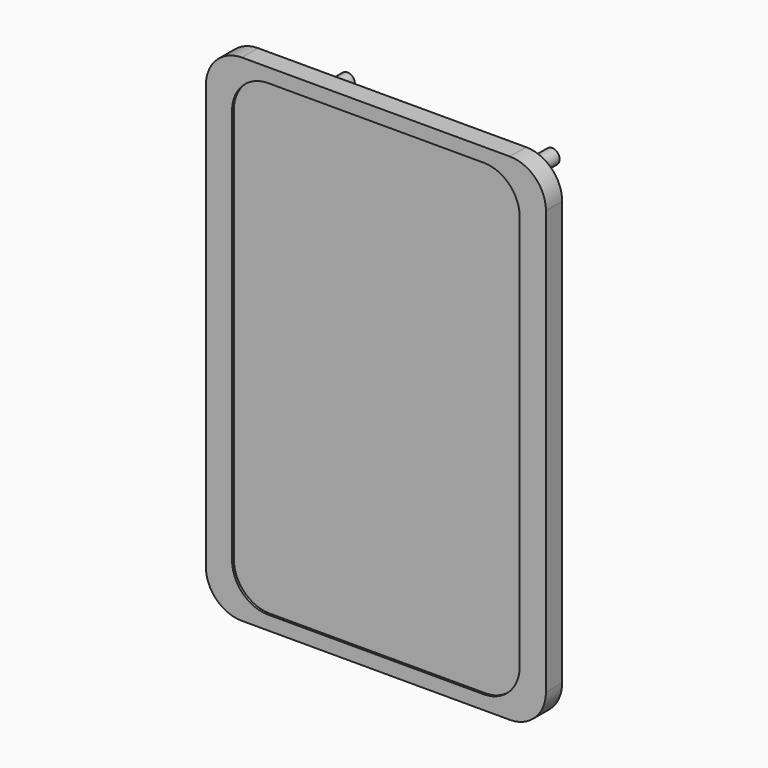
from build123d import *

# Parameters (mm, degrees)
F0_R     = 2.5
F0_W     = 0.95
F0_H     = 30
F0_R_2   = 1.2
F0_R_3   = 0.825
F1_DEPTH = 2
F2_DEPTH = 2
F3_DEPTH = 2.25
F4_DEPTH = 8
F5_DEPTH = 5.5
F6_DEPTH = 3.9


# Not quite as in the source:
# - a feature names something its author has since deleted; it is built from what else it names


with BuildPart() as f1:
    # F0 (on Front) → F1 (new body)
    with BuildSketch(Plane.XZ):
        with BuildLine():
            Line((0, 25), (0, -25))
            Line((0, -25), (11, -25))
            ThreePointArc((11, -25), (13.8284271247, -23.8284271247), (15, -21))
            Line((15, -21), (15, -15))
            Line((15, -15), (15, 15))
            Line((15, 15), (15, 21))
            ThreePointArc((15, 21), (13.8284271247, 23.8284271247), (11, 25))
            Line((11, 25), (0, 25))
        make_face()
        with Locations((11.35, -16.05)):
            Circle(F0_R, mode=Mode.SUBTRACT)
        with Locations((11.35, 22.2)):
            Circle(F0_R, mode=Mode.SUBTRACT)
        with BuildLine():
            Line((-11, -25), (0, -25))
            Line((0, -25), (0, 25))
            Line((0, 25), (-11, 25))
            ThreePointArc((-11, 25), (-13.8284271247, 23.8284271247), (-15, 21))
            Line((-15, 21), (-15, 15))
            Line((-15, 15), (-15, -15))
            Line((-15, -15), (-15, -21))
            ThreePointArc((-15, -21), (-13.8284271247, -23.8284271247), (-11, -25))
        make_face()
        with Locations((-11.35, -16.05)):
            Circle(F0_R, mode=Mode.SUBTRACT)
        with Locations((-11.35, 22.2)):
            Circle(F0_R, mode=Mode.SUBTRACT)
        with BuildLine():
            Line((0, -27.5), (0, -25.95))
            Line((0, -25.95), (-11.95, -25.95))
            ThreePointArc((-11.95, -25.95), (-14.7784271247, -24.7784271247), (-15.95, -21.95))
            Line((-15.95, -21.95), (-15.95, -15))
            Line((-15.95, -15), (-15.95, 15))
            Line((-15.95, 15), (-15.95, 21.95))
            ThreePointArc((-15.95, 21.95), (-14.7784271247, 24.7784271247), (-11.95, 25.95))
            Line((-11.95, 25.95), (0, 25.95))
            Line((0, 25.95), (0, 27.5))
            Line((0, 27.5), (-14.8588332385, 27.5))
            ThreePointArc((-14.8588332385, 27.5), (-17.6872603632, 26.3284271247), (-18.8588332385, 23.5))
            Line((-18.8588332385, 23.5), (-18.8588332385, -23.5))
            ThreePointArc((-18.8588332385, -23.5), (-17.6872603632, -26.3284271247), (-14.8588332385, -27.5))
            Line((-14.8588332385, -27.5), (0, -27.5))
        make_face()
        with BuildLine():
            ThreePointArc((15.95, -21.95), (14.7784271247, -24.7784271247), (11.95, -25.95))
            Line((11.95, -25.95), (0, -25.95))
            Line((0, -25.95), (0, -27.5))
            Line((0, -27.5), (14.8588332385, -27.5))
            ThreePointArc((14.8588332385, -27.5), (17.6872603632, -26.3284271247), (18.8588332385, -23.5))
            Line((18.8588332385, -23.5), (18.8588332385, 23.5))
            ThreePointArc((18.8588332385, 23.5), (17.6872603632, 26.3284271247), (14.8588332385, 27.5))
            Line((14.8588332385, 27.5), (0, 27.5))
            Line((0, 27.5), (0, 25.95))
            Line((0, 25.95), (11.95, 25.95))
            ThreePointArc((11.95, 25.95), (14.7784271247, 24.7784271247), (15.95, 21.95))
            Line((15.95, 21.95), (15.95, 15))
            Line((15.95, 15), (15.95, -15))
            Line((15.95, -15), (15.95, -21.95))
        make_face()
        with Locations((15.475, 0)):
            Rectangle(F0_W, F0_H)
        with Locations((-15.475, 0)):
            Rectangle(F0_W, F0_H)
        with BuildLine():
            Line((-11, 25), (0, 25))
            Line((0, 25), (0, 25.95))
            Line((0, 25.95), (-11.95, 25.95))
            ThreePointArc((-11.95, 25.95), (-14.7784271247, 24.7784271247), (-15.95, 21.95))
            Line((-15.95, 21.95), (-15.95, 15))
            Line((-15.95, 15), (-15, 15))
            Line((-15, 15), (-15, 21))
            ThreePointArc((-15, 21), (-13.8284271247, 23.8284271247), (-11, 25))
        make_face()
        with BuildLine():
            Line((0, 25.95), (0, 25))
            Line((0, 25), (11, 25))
            ThreePointArc((11, 25), (13.8284271247, 23.8284271247), (15, 21))
            Line((15, 21), (15, 15))
            Line((15, 15), (15.95, 15))
            Line((15.95, 15), (15.95, 21.95))
            ThreePointArc((15.95, 21.95), (14.7784271247, 24.7784271247), (11.95, 25.95))
            Line((11.95, 25.95), (0, 25.95))
        make_face()
        with BuildLine():
            Line((0, -25.95), (11.95, -25.95))
            ThreePointArc((11.95, -25.95), (14.7784271247, -24.7784271247), (15.95, -21.95))
            Line((15.95, -21.95), (15.95, -15))
            Line((15.95, -15), (15, -15))
            Line((15, -15), (15, -21))
            ThreePointArc((15, -21), (13.8284271247, -23.8284271247), (11, -25))
            Line((11, -25), (0, -25))
            Line((0, -25), (0, -25.95))
        make_face()
        with BuildLine():
            Line((-11.95, -25.95), (0, -25.95))
            Line((0, -25.95), (0, -25))
            Line((0, -25), (-11, -25))
            ThreePointArc((-11, -25), (-13.8284271247, -23.8284271247), (-15, -21))
            Line((-15, -21), (-15, -15))
            Line((-15, -15), (-15.95, -15))
            Line((-15.95, -15), (-15.95, -21.95))
            ThreePointArc((-15.95, -21.95), (-14.7784271247, -24.7784271247), (-11.95, -25.95))
        make_face()
        with Locations((11.35, -16.05)):
            Circle(F0_R)
        with Locations((11.35, -16.05)):
            Circle(F0_R_2, mode=Mode.SUBTRACT)
        with Locations((-11.35, -16.05)):
            Circle(F0_R)
        with Locations((-11.35, -16.05)):
            Circle(F0_R_2, mode=Mode.SUBTRACT)
        with Locations((11.35, 22.2)):
            Circle(F0_R)
        with Locations((11.35, 22.2)):
            Circle(F0_R_2, mode=Mode.SUBTRACT)
        with Locations((-11.35, 22.2)):
            Circle(F0_R)
        with Locations((-11.35, 22.2)):
            Circle(F0_R_2, mode=Mode.SUBTRACT)
        with Locations((-11.35, -16.05)):
            Circle(F0_R_2)
        with Locations((-11.35, -16.05)):
            Circle(F0_R_3, mode=Mode.SUBTRACT)
        with Locations((11.35, 22.2)):
            Circle(F0_R_2)
        with Locations((11.35, 22.2)):
            Circle(F0_R_3, mode=Mode.SUBTRACT)
        with Locations((-11.35, 22.2)):
            Circle(F0_R_2)
        with Locations((-11.35, 22.2)):
            Circle(F0_R_3, mode=Mode.SUBTRACT)
        with Locations((11.35, -16.05)):
            Circle(F0_R_2)
        with Locations((11.35, -16.05)):
            Circle(F0_R_3, mode=Mode.SUBTRACT)
        with Locations((-11.35, -16.05)):
            Circle(F0_R_3)
        with Locations((11.35, -16.05)):
            Circle(F0_R_3)
        with Locations((11.35, 22.2)):
            Circle(F0_R_3)
        with Locations((-11.35, 22.2)):
            Circle(F0_R_3)
    extrude(amount=F1_DEPTH)

    # F0 (on Front) → F2 (join)
    with BuildSketch(Plane.XZ):
        with BuildLine():
            Line((0, -25.95), (11.95, -25.95))
            ThreePointArc((11.95, -25.95), (14.7784271247, -24.7784271247), (15.95, -21.95))
            Line((15.95, -21.95), (15.95, -15))
            Line((15.95, -15), (15, -15))
            Line((15, -15), (15, -21))
            ThreePointArc((15, -21), (13.8284271247, -23.8284271247), (11, -25))
            Line((11, -25), (0, -25))
            Line((0, -25), (0, -25.95))
        make_face()
        with Locations((15.475, 0)):
            Rectangle(F0_W, F0_H)
        with BuildLine():
            Line((0, 25.95), (0, 25))
            Line((0, 25), (11, 25))
            ThreePointArc((11, 25), (13.8284271247, 23.8284271247), (15, 21))
            Line((15, 21), (15, 15))
            Line((15, 15), (15.95, 15))
            Line((15.95, 15), (15.95, 21.95))
            ThreePointArc((15.95, 21.95), (14.7784271247, 24.7784271247), (11.95, 25.95))
            Line((11.95, 25.95), (0, 25.95))
        make_face()
        with BuildLine():
            Line((-11.95, -25.95), (0, -25.95))
            Line((0, -25.95), (0, -25))
            Line((0, -25), (-11, -25))
            ThreePointArc((-11, -25), (-13.8284271247, -23.8284271247), (-15, -21))
            Line((-15, -21), (-15, -15))
            Line((-15, -15), (-15.95, -15))
            Line((-15.95, -15), (-15.95, -21.95))
            ThreePointArc((-15.95, -21.95), (-14.7784271247, -24.7784271247), (-11.95, -25.95))
        make_face()
        with Locations((-15.475, 0)):
            Rectangle(F0_W, F0_H)
        with BuildLine():
            Line((-11, 25), (0, 25))
            Line((0, 25), (0, 25.95))
            Line((0, 25.95), (-11.95, 25.95))
            ThreePointArc((-11.95, 25.95), (-14.7784271247, 24.7784271247), (-15.95, 21.95))
            Line((-15.95, 21.95), (-15.95, 15))
            Line((-15.95, 15), (-15, 15))
            Line((-15, 15), (-15, 21))
            ThreePointArc((-15, 21), (-13.8284271247, 23.8284271247), (-11, 25))
        make_face()
    extrude(amount=-F2_DEPTH)

    # F0 (on Front) → F3 (join)
    with BuildSketch(Plane.XZ):
        with BuildLine():
            ThreePointArc((15.95, -21.95), (14.7784271247, -24.7784271247), (11.95, -25.95))
            Line((11.95, -25.95), (0, -25.95))
            Line((0, -25.95), (0, -27.5))
            Line((0, -27.5), (14.8588332385, -27.5))
            ThreePointArc((14.8588332385, -27.5), (17.6872603632, -26.3284271247), (18.8588332385, -23.5))
            Line((18.8588332385, -23.5), (18.8588332385, 23.5))
            ThreePointArc((18.8588332385, 23.5), (17.6872603632, 26.3284271247), (14.8588332385, 27.5))
            Line((14.8588332385, 27.5), (0, 27.5))
            Line((0, 27.5), (0, 25.95))
            Line((0, 25.95), (11.95, 25.95))
            ThreePointArc((11.95, 25.95), (14.7784271247, 24.7784271247), (15.95, 21.95))
            Line((15.95, 21.95), (15.95, 15))
            Line((15.95, 15), (15.95, -15))
            Line((15.95, -15), (15.95, -21.95))
        make_face()
        with BuildLine():
            Line((0, -27.5), (0, -25.95))
            Line((0, -25.95), (-11.95, -25.95))
            ThreePointArc((-11.95, -25.95), (-14.7784271247, -24.7784271247), (-15.95, -21.95))
            Line((-15.95, -21.95), (-15.95, -15))
            Line((-15.95, -15), (-15.95, 15))
            Line((-15.95, 15), (-15.95, 21.95))
            ThreePointArc((-15.95, 21.95), (-14.7784271247, 24.7784271247), (-11.95, 25.95))
            Line((-11.95, 25.95), (0, 25.95))
            Line((0, 25.95), (0, 27.5))
            Line((0, 27.5), (-14.8588332385, 27.5))
            ThreePointArc((-14.8588332385, 27.5), (-17.6872603632, 26.3284271247), (-18.8588332385, 23.5))
            Line((-18.8588332385, 23.5), (-18.8588332385, -23.5))
            ThreePointArc((-18.8588332385, -23.5), (-17.6872603632, -26.3284271247), (-14.8588332385, -27.5))
            Line((-14.8588332385, -27.5), (0, -27.5))
        make_face()
    extrude(amount=F3_DEPTH)

    # F0 (on Front) → F4 (join)
    with BuildSketch(Plane.XZ):
        with Locations((11.35, -16.05)):
            Circle(F0_R_3)
        with Locations((-11.35, -16.05)):
            Circle(F0_R_3)
        with Locations((-11.35, 22.2)):
            Circle(F0_R_3)
        with Locations((11.35, 22.2)):
            Circle(F0_R_3)
    extrude(amount=-F4_DEPTH)

    # F0 (on Front) → F5 (join)
    with BuildSketch(Plane.XZ):
        with Locations((11.35, -16.05)):
            Circle(F0_R_2)
        with Locations((11.35, -16.05)):
            Circle(F0_R_3, mode=Mode.SUBTRACT)
        with Locations((-11.35, -16.05)):
            Circle(F0_R_2)
        with Locations((-11.35, -16.05)):
            Circle(F0_R_3, mode=Mode.SUBTRACT)
        with Locations((-11.35, 22.2)):
            Circle(F0_R_2)
        with Locations((-11.35, 22.2)):
            Circle(F0_R_3, mode=Mode.SUBTRACT)
        with Locations((11.35, 22.2)):
            Circle(F0_R_2)
        with Locations((11.35, 22.2)):
            Circle(F0_R_3, mode=Mode.SUBTRACT)
    extrude(amount=-F5_DEPTH)

    # F0 (on Front) → F6 (join)
    with BuildSketch(Plane.XZ):
        with Locations((11.35, 22.2)):
            Circle(F0_R)
        with Locations((11.35, 22.2)):
            Circle(F0_R_2, mode=Mode.SUBTRACT)
        with Locations((-11.35, 22.2)):
            Circle(F0_R)
        with Locations((-11.35, 22.2)):
            Circle(F0_R_2, mode=Mode.SUBTRACT)
        with Locations((11.35, -16.05)):
            Circle(F0_R)
        with Locations((11.35, -16.05)):
            Circle(F0_R_2, mode=Mode.SUBTRACT)
        with Locations((-11.35, -16.05)):
            Circle(F0_R)
        with Locations((-11.35, -16.05)):
            Circle(F0_R_2, mode=Mode.SUBTRACT)
    extrude(amount=-F6_DEPTH)


solid = f1.part
